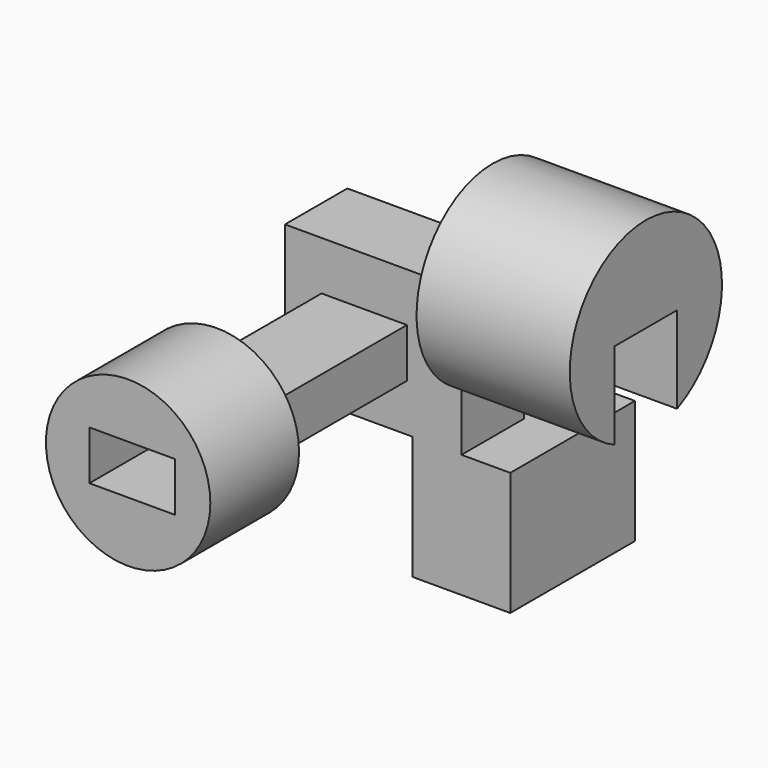
from build123d import *

# Parameters (mm, degrees)
F0_W        = 113.259896636
F0_H        = 93.3482274413
F1_DEPTH    = 25
F2_W        = 54.8066571355
F2_H        = 31.5346177667
F3_DEPTH    = 115.0439456105
F1_FACE_W   = 113.259896636
F1_FACE_H   = 93.3482274413
F1_FACE_W_2 = 54.8066571355
F1_FACE_H_2 = 31.5346177667
F4_W        = 54.8066571355
F4_H        = 31.5346177667
F5_DEPTH    = 25
F6_R        = 52.7555643641
F6_W        = 54.8066571355
F6_H        = 31.5346177667
F7_DEPTH    = 71.1605325341
F8_W        = 62.6089163125
F8_H        = 100
F9_DEPTH    = 79.2002081871
F14_DEPTH   = 98.3245372772


# Not quite as in the source:
# - the program builds the solid bodies; features that only make, move or delete a surface that nothing else refers to are left out


with BuildPart() as f1:
    # F0 (on Front) → F1 (new body)
    with BuildSketch(Plane.XZ):
        Rectangle(F0_W, F0_H)
    extrude(amount=F1_DEPTH)

    # F2 (on face) → F3 (join)
    with BuildSketch(Plane.XZ.offset(25)):
        with Locations((-5.7783313096, -0.4667351022)):
            Rectangle(F2_W, F2_H)
    extrude(amount=F3_DEPTH)

    # F1_face (on face) + F4 (on face) → F5 (join)
    with BuildSketch(Plane.XZ.offset(25)):
        Rectangle(F1_FACE_W, F1_FACE_H)
        with Locations((-5.7783313096, -0.4667351022)):
            Rectangle(F1_FACE_W_2, F1_FACE_H_2, mode=Mode.SUBTRACT)
    with BuildSketch(Plane.XZ.offset(140.0439456105)):
        with Locations((-5.7783313096, -0.4667351022)):
            Rectangle(F4_W, F4_H)
    extrude(amount=F5_DEPTH)

    # F8 (on face) → F9 (join)
    with BuildSketch(Plane(origin=(0, 0, -46.6741137207), x_dir=(1, 0, 0), z_dir=(0, 0, -1))):
        with Locations((56.629948318, 0)):
            Rectangle(F8_W, F8_H)
    extrude(amount=F9_DEPTH)


with BuildPart() as f7:
    # F6 (on face) → F7 (new body)
    with BuildSketch(Plane.XZ.offset(165.0439456105)):
        with Locations((-8.3341598511, -2.1851621568)):
            Circle(F6_R)
        with Locations((-5.7783313096, -0.4667351022)):
            Rectangle(F6_W, F6_H, mode=Mode.SUBTRACT)
    extrude(amount=F7_DEPTH)


with BuildPart() as f14:
    # F13 (on face) → F14 (new body)
    with BuildSketch(Plane.YZ.offset(56.629948318)):
        with BuildLine():
            ThreePointArc((0, -9.0233932707), (26.2517549134, 13.5007825139), (36.0508991339, 46.6741137207))
            ThreePointArc((36.0508991339, 46.6741137207), (-58.1733312068, 97.925868634), (-50, -9.0233932707))
            Line((-50, -9.0233932707), (-50, 46.6741137207))
            Line((-50, 46.6741137207), (0, 46.6741137207))
            Line((0, 46.6741137207), (0, -9.0233932707))
        make_face()
    extrude(amount=F14_DEPTH)


solid = Compound([f1.part, f7.part, f14.part])
